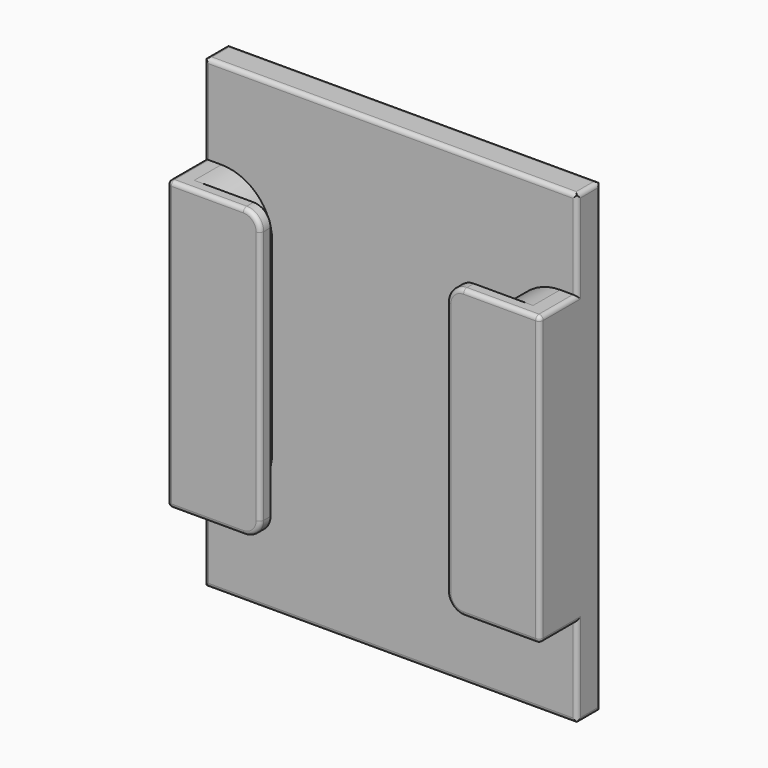
from build123d import *

# Parameters (mm, degrees)
F0_W        = 22
F0_H        = 55
F1_DEPTH    = 3.5
F3_DEPTH    = 4
F5_DEPTH    = 1.5
F6_R        = 0.5
F8_T1_DEPTH = 45.5


# Not quite as in the source:
# - a fillet or chamfer that OpenCascade refuses, or shapes differently, is made with other operations: its cross-section is extruded or revolved along the edge and cut away or added


with BuildPart() as f1:
    # F0 (on Front) → F1 (new body)
    with BuildSketch(Plane.XZ):
        with Locations((11, -27.5)):
            Rectangle(F0_W, F0_H)
    extrude(amount=F1_DEPTH)

    # F2 (on face) → F3 (join)
    with BuildSketch(Plane.XZ.offset(3.5)):
        with BuildLine():
            Line((2, -10.5), (0, -10.5))
            Line((0, -10.5), (0, -44.5))
            Line((0, -44.5), (2, -44.5))
            ThreePointArc((2, -44.5), (6.2426406871, -42.7426406871), (8, -38.5))
            Line((8, -38.5), (8, -16.5))
            ThreePointArc((8, -16.5), (6.2426406871, -12.2573593129), (2, -10.5))
        make_face()
    extrude(amount=F3_DEPTH)

    # F4 (on face) → F5 (join)
    with BuildSketch(Plane.XZ.offset(7.5)):
        with BuildLine():
            Line((9, -10.5), (0, -10.5))
            Line((0, -10.5), (0, -44.5))
            Line((0, -44.5), (9, -44.5))
            ThreePointArc((9, -44.5), (10.4142135624, -43.9142135624), (11, -42.5))
            Line((11, -42.5), (11, -12.5))
            ThreePointArc((11, -12.5), (10.4142135624, -11.0857864376), (9, -10.5))
        make_face()
    extrude(amount=F5_DEPTH)

    # F6
    f6_edges = [f1.edges().sort_by_distance(p)[0] for p in [
        (10.414214, -9, -11.085786),
        (4.5, -9, -10.5),
        (0, -9, -27.5),
        (4.5, -9, -44.5),
        (10.414214, -9, -43.914214),
        (11, -9, -27.5),
        (0, -1.75, 0),
        (0, -3.5, -5.25),
        (0, -6.25, -10.5),
        (0, -6.25, -44.5),
        (0, -3.5, -49.75),
        (0, -1.75, -55),
        (0, 0, -27.5),
    ]]
    fillet(f6_edges, radius=F6_R)

    # F7: F1 across face


with BuildPart() as f1_1:
    add(f1.part)
    add(f1.part.mirror(Plane(origin=(22, -1.75, -27.5), x_dir=(0, 1, 0), z_dir=(1, 0, 0))))

    # F8: fillet of radius 0.5 on 8 edges, made by hand

    # F8_s2 → F8_t1 (cut)
    with BuildSketch(Plane.YZ.offset(-0.75)):
        with BuildLine():
            ThreePointArc((-3, -55), (-3.3535533906, -54.8535533906), (-3.5, -54.5))
            Line((-3.5, -54.5), (-3.5, -55))
            Line((-3.5, -55), (-3, -55))
        make_face()
        with BuildLine():
            ThreePointArc((-0.5, -55), (-0.1464466094, -54.8535533906), (0, -54.5))
            Line((0, -54.5), (0, -55))
            Line((0, -55), (-0.5, -55))
        make_face()
        with BuildLine():
            ThreePointArc((-0.5, 0), (-0.1464466094, -0.1464466094), (0, -0.5))
            Line((0, -0.5), (0, 0))
            Line((0, 0), (-0.5, 0))
        make_face()
        with BuildLine():
            ThreePointArc((-3, 0), (-3.3535533906, -0.1464466094), (-3.5, -0.5))
            Line((-3.5, -0.5), (-3.5, 0))
            Line((-3.5, 0), (-3, 0))
        make_face()
    extrude(amount=F8_T1_DEPTH, mode=Mode.SUBTRACT)


solid = f1_1.part
